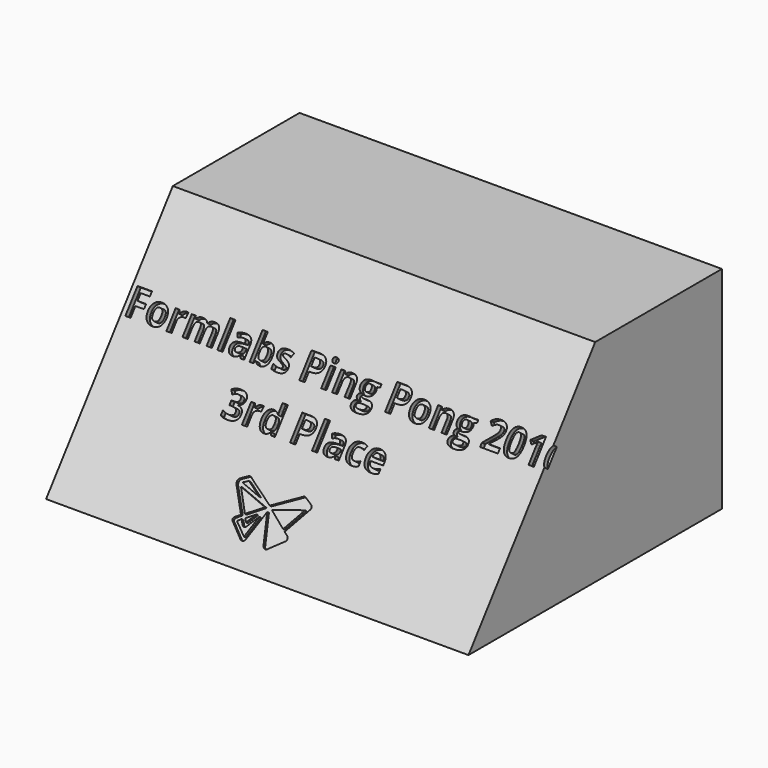
from build123d import *

# Parameters (mm, degrees)
F0_W         = 101.6
F0_H         = 76.2
F1_DEPTH     = 50.8
F3_DEPTH     = 101.601
F4_T         = -2.54
F5_TEXT_SIZE = 8.5353903059
F6_DEPTH     = 1.27
F8_DEPTH     = 0.635
F9_TEXT_SIZE = 5.3735863831
F10_DEPTH    = 1.27


# Not quite as in the source:
# - Text() gives the source's letters only with a copy of the font that has no kerning and outlines rounded to 1/6400 em; it was checked with that copy


with BuildPart() as f1:
    # F0 (on Top) → F1 (new body)
    with BuildSketch(Plane.XY):
        with Locations((16.9333308506, 38.1)):
            Rectangle(F0_W, F0_H)
    extrude(amount=F1_DEPTH)

    # F2 (on face) → F3 (cut, through all)
    with BuildSketch(Plane.YZ.offset(67.7333308506)):
        Polygon((0, 50.8), (0, 0), (38.1, 50.8), align=None)
    extrude(amount=-F3_DEPTH, mode=Mode.SUBTRACT)

    # F4
    f4_openings = [f1.faces().sort_by_distance(p)[0] for p in [
        (16.933331, 38.1, 0),
    ]]
    offset(amount=F4_T, openings=f4_openings)

    # F5 (on face) → F6 (cut)
    with BuildSketch(Plane(origin=(0, 0, 0), x_dir=(1, 0, 0), z_dir=(0, -0.8, 0.6))):
        with Locations((-33.5582504049, 37.4789871275)):
            Text('Formlabs Ping Pong 2016', F5_TEXT_SIZE, font='Open Sans', font_style=FontStyle.BOLD, text_align=(TextAlign.LEFT, TextAlign.BOTTOM))
        with Locations((-4.7259686827, 25.8708563116)):
            Text('3rd Place', F5_TEXT_SIZE, font='Open Sans', font_style=FontStyle.BOLD, text_align=(TextAlign.LEFT, TextAlign.BOTTOM))
    extrude(amount=-F6_DEPTH, mode=Mode.SUBTRACT)

    # F7 (on face) → F8 (cut)
    with BuildSketch(Plane(origin=(0, 0, 0), x_dir=(1, 0, 0), z_dir=(0, -0.8, 0.6))):
        with BuildLine():
            Line((13.4837115183, 13.4272510186), (7.3560709134, 17.118493095))
            ThreePointArc((7.3560709134, 17.118493095), (6.9598628009, 17.3219317084), (6.5232547931, 17.2339454293))
            Line((6.5232547931, 17.2339454293), (5.0372248515, 16.3523033261))
            ThreePointArc((5.0372248515, 16.3523033261), (4.5941037589, 15.7553422177), (4.7088782303, 15.0208044797))
            Line((4.7088782303, 15.0208044797), (8.2500472502, 9.9444482787))
            Line((8.2500472502, 9.9444482787), (7.0838008274, 9.1308970741))
            ThreePointArc((7.0838008274, 9.1308970741), (6.8475814061, 8.6456949987), (7.1361442097, 8.1896772608))
            Line((7.1361442097, 8.1896772608), (10.2178193629, 5.5576669984))
            ThreePointArc((10.2178193629, 5.5576669984), (10.8682715637, 5.4446336831), (11.3433087245, 5.9031140991))
            Line((11.3433087245, 5.9031140991), (13.5008823127, 12.1355671436))
            Line((13.5008823127, 12.1355671436), (15.5845545232, 5.9314654209))
            ThreePointArc((15.5845545232, 5.9314654209), (15.9616371116, 5.4979932508), (16.5347233415, 5.4572308436))
            Line((16.5347233415, 5.4572308436), (19.7310019284, 8.081631735))
            ThreePointArc((19.7310019284, 8.081631735), (20.041796176, 8.6354321435), (19.7362490992, 9.1921447629))
            Line((19.7362490992, 9.1921447629), (18.8143051114, 9.7729407743))
            Line((18.8143051114, 9.7729407743), (22.2590983821, 15.2411368069))
            ThreePointArc((22.2590983821, 15.2411368069), (22.3842901343, 15.813418361), (22.0345240086, 16.2833575159))
            Line((22.0345240086, 16.2833575159), (20.3393120319, 17.2168835998))
            ThreePointArc((20.3393120319, 17.2168835998), (19.9693319663, 17.2853947372), (19.6317466821, 17.1192165172))
            Line((19.6317466821, 17.1192165172), (13.4837115183, 13.4272510186))
        make_face()
        with BuildLine():
            Line((10.2651705965, 8.0516058952), (12.2502879319, 10.7989438046))
            Line((12.2502879319, 10.7989438046), (10.7283759862, 6.2629207969))
            Line((10.7283759862, 6.2629207969), (7.9214246944, 8.5824187845))
            Line((7.9214246944, 8.5824187845), (8.7465365849, 9.2327181414))
            Line((8.7465365849, 9.2327181414), (9.4287740067, 8.2547133788))
            ThreePointArc((9.4287740067, 8.2547133788), (9.8085458541, 7.9949195314), (10.2651705965, 8.0516058952))
        make_face(mode=Mode.SUBTRACT)
        Polygon((9.4586731866, 9.6149612218), (11.4831300452, 11.0469274223), (9.9453385919, 8.9157661423), align=None, mode=Mode.SUBTRACT)
        Polygon((5.8720999334, 14.8942405851), (12.6240206882, 12.8366881981), (8.9787328616, 10.3465225548), align=None, mode=Mode.SUBTRACT)
        Polygon((5.7934536599, 15.7347135246), (7.0594344288, 16.4298992604), (10.5455731973, 14.3083883449), align=None, mode=Mode.SUBTRACT)
        Polygon((14.2554277554, 12.8213027492), (21.3006008416, 14.9052804336), (18.2668808848, 10.1485736668), align=None, mode=Mode.SUBTRACT)
    extrude(amount=-F8_DEPTH, mode=Mode.SUBTRACT)

    # F9 (on face) → F10 (cut)
    with BuildSketch(Plane.XZ.offset(-73.66)):
        with Locations((-21.9453405589, 9.4390390441)):
            Text('Designed & Printed by David Liu', F9_TEXT_SIZE, font='Open Sans', text_align=(TextAlign.LEFT, TextAlign.BOTTOM))
    extrude(amount=-F10_DEPTH, mode=Mode.SUBTRACT)


solid = f1.part
